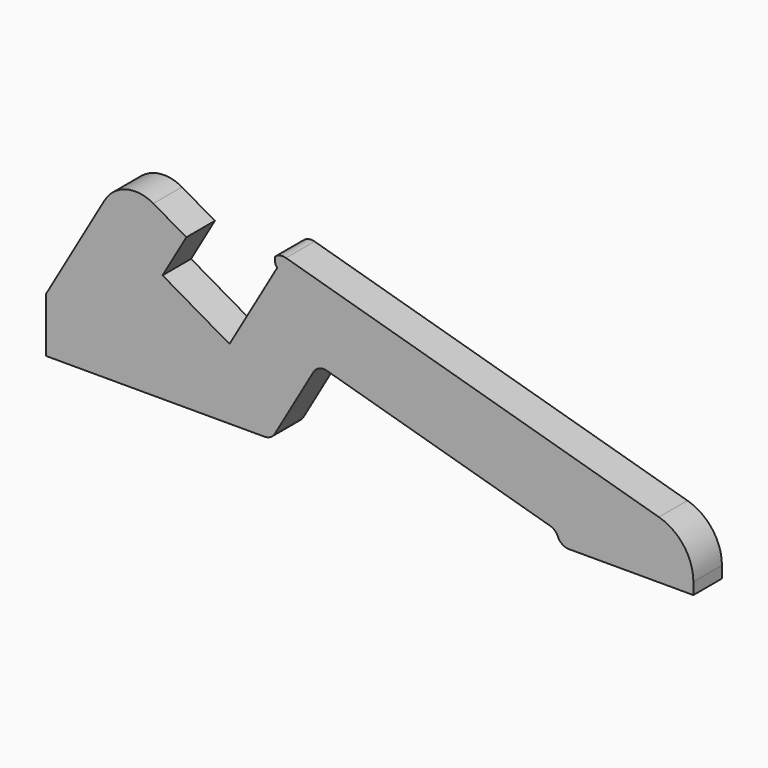
from build123d import *

# Parameters (mm, degrees)
F1_DEPTH    = 3.81
F2_T1_DEPTH = 8.770689479
F2_T3_DEPTH = 9.6298711326
F3_R        = 3.81
F4_R        = 5.08
F5_R        = 1.27
F6_R        = 1.27


# Not quite as in the source:
# - a fillet or chamfer that OpenCascade refuses, or shapes differently, is made with other operations: its cross-section is extruded or revolved along the edge and cut away or added


with BuildPart() as f1:
    # F0 (on Front) → F1 (new body)
    with BuildSketch(Plane.XZ):
        Polygon((0, 5.842), (0, 0), (24.0501028134, 0), (29.035013032, 8.6341177699), (54.7257371953, 1.27), (54.7257371953, 0), (69.088, 0), (69.088, 5.08), (24.657370278, 17.8158181024), (23.9974589203, 16.6728181024), (24.657370278, 16.2918181024), (19.577370278, 7.493), (12.4283305697, 11.6205), (14.9683305697, 16.0199090512), (8.1492465403, 19.9569090512), align=None)
    extrude(amount=F1_DEPTH)

    # F2: fillet of radius 1.27 on 2 edges, made by hand

    # F2_s2 → F2_t1 (cut)
    with BuildSketch(Plane.XZ.offset(-2.4803447395)):
        with BuildLine():
            ThreePointArc((25.6110997962, 17.5424362994), (24.7853486084, 17.4991029103), (24.16130133, 16.9566014806))
            Line((24.16130133, 16.9566014806), (24.657370278, 17.8158181024))
            Line((24.657370278, 17.8158181024), (25.6110997962, 17.5424362994))
        make_face()
    extrude(amount=F2_T1_DEPTH, mode=Mode.SUBTRACT)

    # F2_s4 → F2_t3 (cut)
    with BuildSketch(Plane.XZ.offset(-2.9099355663)):
        with BuildLine():
            ThreePointArc((24.5794460335, 17.680849352), (24.4112920489, 16.9747145746), (24.657370278, 16.2918181024))
            Line((24.657370278, 16.2918181024), (23.9974589203, 16.6728181024))
            Line((23.9974589203, 16.6728181024), (24.5794460335, 17.680849352))
        make_face()
    extrude(amount=F2_T3_DEPTH, mode=Mode.SUBTRACT)

    # F3
    f3_edges = [f1.edges().sort_by_distance(p)[0] for p in [
        (8.149247, -1.905, 19.956909),
    ]]
    fillet(f3_edges, radius=F3_R)

    # F4
    f4_edges = [f1.edges().sort_by_distance(p)[0] for p in [
        (69.088, -1.905, 5.08),
    ]]
    fillet(f4_edges, radius=F4_R)

    # F5
    f5_edges = [f1.edges().sort_by_distance(p)[0] for p in [
        (29.035013, -1.905, 8.634118),
        (24.050103, -1.905, 0),
        (54.725737, -1.905, 1.27),
    ]]
    fillet(f5_edges, radius=F5_R)

    # F6
    f6_edges = [f1.edges().sort_by_distance(p)[0] for p in [
        (54.725737, -1.905, 0),
    ]]
    fillet(f6_edges, radius=F6_R)


solid = f1.part
